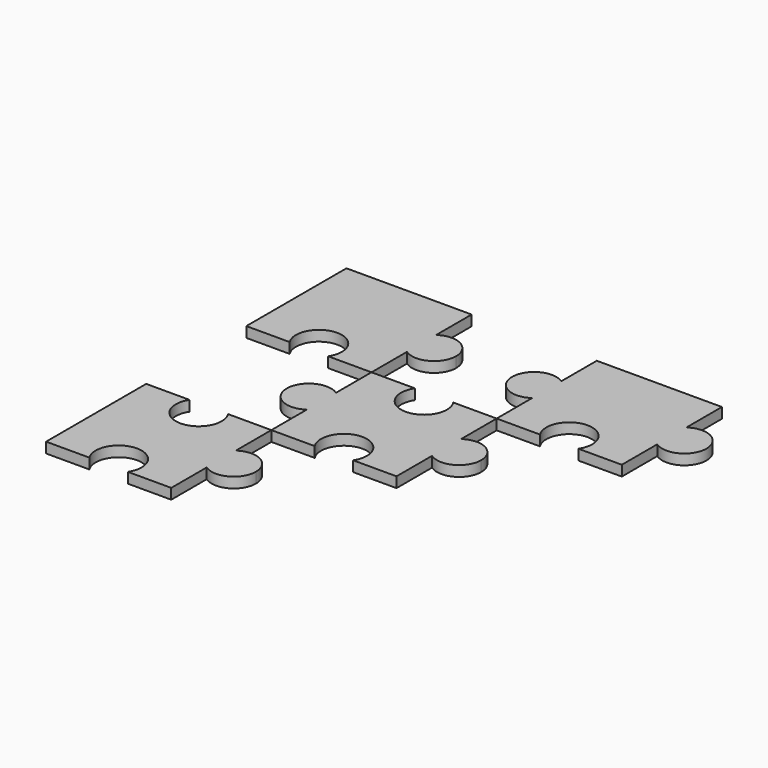
from build123d import *

# Parameters (mm, degrees)
F1_DEPTH = 2.5
F2_DEPTH = 2.5
F3_DEPTH = 2.5
F4_DEPTH = 2.5
F5_ANGLE = 45
F7_ANGLE = -45


# Not quite as in the source:
# - a pattern or mirror of a feature is missing from the dataset's text; its kind, count and spacing are read off the source's solid
# - a feature names something its author has since deleted; it is built from what else it names


with BuildPart() as f1:
    # F0 (on Top) → F1 (new body)
    with BuildSketch(Plane.XY):
        with BuildLine():
            Line((15, 4.6097722286), (15, 15))
            Line((15, 15), (4.6097722286, 15))
            ThreePointArc((4.6097722286, 15), (5.2727482046, 13.564648961), (5.5, 12))
            ThreePointArc((5.5, 12), (-1.564648961, 6.7272517954), (-4.6097722286, 15))
            Line((-4.6097722286, 15), (-15, 15))
            Line((-15, 15), (-15, 4.6097722286))
            ThreePointArc((-15, 4.6097722286), (-9.3779778796, 4.8347699015), (-6.5, 0))
            ThreePointArc((-6.5, 0), (-9.3779778796, -4.8347699015), (-15, -4.6097722286))
            Line((-15, -4.6097722286), (-15, -15))
            Line((-15, -15), (-4.6097722286, -15))
            ThreePointArc((-4.6097722286, -15), (-1.564648961, -6.7272517954), (5.5, -12))
            ThreePointArc((5.5, -12), (5.2727482046, -13.564648961), (4.6097722286, -15))
            Line((4.6097722286, -15), (15, -15))
            Line((15, -15), (15, -4.6097722286))
            ThreePointArc((15, -4.6097722286), (6.5, 0), (15, 4.6097722286))
        make_face()
        with BuildLine():
            ThreePointArc((5.5, 12), (5.2727482046, 13.564648961), (4.6097722286, 15))
            Line((4.6097722286, 15), (4.369210455, 15))
            ThreePointArc((4.369210455, 15), (5.0619569048, 13.5705388547), (5.3, 12))
            ThreePointArc((5.3, 12), (-1.5705388547, 6.9380430952), (-4.369210455, 15))
            Line((-4.369210455, 15), (-4.6097722286, 15))
            ThreePointArc((-4.6097722286, 15), (-1.564648961, 6.7272517954), (5.5, 12))
        make_face()
        with BuildLine():
            ThreePointArc((15.18, 4.4874937326), (15.0893990769, 4.4292665608), (15, 4.369210455))
            ThreePointArc((15, 4.369210455), (16.6898827277, 2.4688053791), (17.3, 0))
            ThreePointArc((17.3, 0), (16.6898827277, -2.4688053791), (15, -4.369210455))
            ThreePointArc((15, -4.369210455), (15.0893990769, -4.4292665608), (15.18, -4.4874937326))
            ThreePointArc((15.18, -4.4874937326), (16.8856934001, -2.5258661881), (17.5, 0))
            ThreePointArc((17.5, 0), (16.8856934001, 2.5258661881), (15.18, 4.4874937326))
        make_face()
        with BuildLine():
            ThreePointArc((-6.7, 0), (-9.5311946209, 4.6898827277), (-15, 4.369210455))
            Line((-15, 4.369210455), (-15, -4.369210455))
            ThreePointArc((-15, -4.369210455), (-9.5311946209, -4.6898827277), (-6.7, 0))
        make_face()
        with BuildLine():
            ThreePointArc((5.3, 12), (5.0619569048, 13.5705388547), (4.369210455, 15))
            Line((4.369210455, 15), (-4.369210455, 15))
            ThreePointArc((-4.369210455, 15), (-1.5705388547, 6.9380430952), (5.3, 12))
        make_face()
        with BuildLine():
            ThreePointArc((14.82, -4.4874937326), (12.5, 0), (14.82, 4.4874937326))
            ThreePointArc((14.82, 4.4874937326), (6.7, 0), (14.82, -4.4874937326))
        make_face()
        with BuildLine():
            Line((15, -4.369210455), (15, 4.369210455))
            ThreePointArc((15, 4.369210455), (12.7, 0), (15, -4.369210455))
        make_face()
        with BuildLine():
            ThreePointArc((17.3, 0), (16.6898827277, 2.4688053791), (15, 4.369210455))
            Line((15, 4.369210455), (15, -4.369210455))
            ThreePointArc((15, -4.369210455), (16.6898827277, -2.4688053791), (17.3, 0))
        make_face()
        with BuildLine():
            ThreePointArc((23.3, 0), (20.5635912311, 4.6387498316), (15.18, 4.4874937326))
            ThreePointArc((15.18, 4.4874937326), (16.8856934001, 2.5258661881), (17.5, 0))
            ThreePointArc((17.5, 0), (16.8856934001, -2.5258661881), (15.18, -4.4874937326))
            ThreePointArc((15.18, -4.4874937326), (20.5635912311, -4.6387498316), (23.3, 0))
        make_face()
        with BuildLine():
            ThreePointArc((15, -4.369210455), (12.7, 0), (15, 4.369210455))
            ThreePointArc((15, 4.369210455), (14.9106009231, 4.4292665608), (14.82, 4.4874937326))
            ThreePointArc((14.82, 4.4874937326), (12.5, 0), (14.82, -4.4874937326))
            ThreePointArc((14.82, -4.4874937326), (14.9106009231, -4.4292665608), (15, -4.369210455))
        make_face()
        with BuildLine():
            ThreePointArc((-6.5, 0), (-9.3779778796, 4.8347699015), (-15, 4.6097722286))
            Line((-15, 4.6097722286), (-15, 4.369210455))
            ThreePointArc((-15, 4.369210455), (-9.5311946209, 4.6898827277), (-6.7, 0))
            ThreePointArc((-6.7, 0), (-9.5311946209, -4.6898827277), (-15, -4.369210455))
            Line((-15, -4.369210455), (-15, -4.6097722286))
            ThreePointArc((-15, -4.6097722286), (-9.3779778796, -4.8347699015), (-6.5, 0))
        make_face()
        with BuildLine():
            ThreePointArc((14.82, 4.4874937326), (14.9093952036, 4.5495232709), (15, 4.6097722286))
            ThreePointArc((15, 4.6097722286), (6.5, 0), (15, -4.6097722286))
            ThreePointArc((15, -4.6097722286), (14.9093952036, -4.5495232709), (14.82, -4.4874937326))
            ThreePointArc((14.82, -4.4874937326), (6.7, 0), (14.82, 4.4874937326))
        make_face()
        with BuildLine():
            Line((15, 4.369210455), (15, 4.6097722286))
            ThreePointArc((15, 4.6097722286), (14.9093952036, 4.5495232709), (14.82, 4.4874937326))
            ThreePointArc((14.82, 4.4874937326), (14.9106009231, 4.4292665608), (15, 4.369210455))
        make_face()
        with BuildLine():
            ThreePointArc((14.82, -4.4874937326), (14.9093952036, -4.5495232709), (15, -4.6097722286))
            Line((15, -4.6097722286), (15, -4.369210455))
            ThreePointArc((15, -4.369210455), (14.9106009231, -4.4292665608), (14.82, -4.4874937326))
        make_face()
    extrude(amount=F1_DEPTH)


with BuildPart() as f2:
    # F0 (on Top) → F2 (new body)
    with BuildSketch(Plane.XY):
        with BuildLine():
            ThreePointArc((44.82, -4.4874937326), (42.5, 0), (44.82, 4.4874937326))
            ThreePointArc((44.82, 4.4874937326), (36.7, 0), (44.82, -4.4874937326))
        make_face()
        with BuildLine():
            Line((45, -4.369210455), (45, 4.369210455))
            ThreePointArc((45, 4.369210455), (42.7, 0), (45, -4.369210455))
        make_face()
        with BuildLine():
            ThreePointArc((45, -4.369210455), (42.7, 0), (45, 4.369210455))
            ThreePointArc((45, 4.369210455), (44.9106009231, 4.4292665608), (44.82, 4.4874937326))
            ThreePointArc((44.82, 4.4874937326), (42.5, 0), (44.82, -4.4874937326))
            ThreePointArc((44.82, -4.4874937326), (44.9106009231, -4.4292665608), (45, -4.369210455))
        make_face()
        with BuildLine():
            ThreePointArc((47.3, 0), (46.6898827277, 2.4688053791), (45, 4.369210455))
            Line((45, 4.369210455), (45, -4.369210455))
            ThreePointArc((45, -4.369210455), (46.6898827277, -2.4688053791), (47.3, 0))
        make_face()
        with BuildLine():
            ThreePointArc((47.5, 0), (46.8856934001, 2.5258661881), (45.18, 4.4874937326))
            ThreePointArc((45.18, 4.4874937326), (45.0893990769, 4.4292665608), (45, 4.369210455))
            ThreePointArc((45, 4.369210455), (46.6898827277, 2.4688053791), (47.3, 0))
            ThreePointArc((47.3, 0), (46.6898827277, -2.4688053791), (45, -4.369210455))
            ThreePointArc((45, -4.369210455), (45.0893990769, -4.4292665608), (45.18, -4.4874937326))
            ThreePointArc((45.18, -4.4874937326), (46.8856934001, -2.5258661881), (47.5, 0))
        make_face()
        with BuildLine():
            ThreePointArc((53.3, 0), (50.5635912311, 4.6387498316), (45.18, 4.4874937326))
            ThreePointArc((45.18, 4.4874937326), (46.8856934001, 2.5258661881), (47.5, 0))
            ThreePointArc((47.5, 0), (46.8856934001, -2.5258661881), (45.18, -4.4874937326))
            ThreePointArc((45.18, -4.4874937326), (50.5635912311, -4.6387498316), (53.3, 0))
        make_face()
        with BuildLine():
            ThreePointArc((53.5, 0), (50.6220221204, 4.8347699015), (45, 4.6097722286))
            ThreePointArc((45, 4.6097722286), (45.0906047964, 4.5495232709), (45.18, 4.4874937326))
            ThreePointArc((45.18, 4.4874937326), (50.5635912311, 4.6387498316), (53.3, 0))
            ThreePointArc((53.3, 0), (50.5635912311, -4.6387498316), (45.18, -4.4874937326))
            ThreePointArc((45.18, -4.4874937326), (45.0906047964, -4.5495232709), (45, -4.6097722286))
            ThreePointArc((45, -4.6097722286), (50.6220221204, -4.8347699015), (53.5, 0))
        make_face()
        with BuildLine():
            Line((55.3902277714, 15), (45, 15))
            Line((45, 15), (45, 4.6097722286))
            ThreePointArc((45, 4.6097722286), (50.6220221204, 4.8347699015), (53.5, 0))
            ThreePointArc((53.5, 0), (50.6220221204, -4.8347699015), (45, -4.6097722286))
            Line((45, -4.6097722286), (45, -15))
            Line((45, -15), (55.3902277714, -15))
            ThreePointArc((55.3902277714, -15), (58.435351039, -6.7272517954), (65.5, -12))
            ThreePointArc((65.5, -12), (65.2727482046, -13.564648961), (64.6097722286, -15))
            Line((64.6097722286, -15), (75, -15))
            Line((75, -15), (75, -4.6097722286))
            ThreePointArc((75, -4.6097722286), (66.5, 0), (75, 4.6097722286))
            Line((75, 4.6097722286), (75, 15))
            Line((75, 15), (64.6097722286, 15))
            ThreePointArc((64.6097722286, 15), (65.2727482046, 13.564648961), (65.5, 12))
            ThreePointArc((65.5, 12), (58.435351039, 6.7272517954), (55.3902277714, 15))
        make_face()
        with BuildLine():
            ThreePointArc((45.18, 4.4874937326), (45.0906047964, 4.5495232709), (45, 4.6097722286))
            Line((45, 4.6097722286), (45, 4.369210455))
            ThreePointArc((45, 4.369210455), (45.0893990769, 4.4292665608), (45.18, 4.4874937326))
        make_face()
        with BuildLine():
            Line((45, -4.369210455), (45, -4.6097722286))
            ThreePointArc((45, -4.6097722286), (45.0906047964, -4.5495232709), (45.18, -4.4874937326))
            ThreePointArc((45.18, -4.4874937326), (45.0893990769, -4.4292665608), (45, -4.369210455))
        make_face()
        with BuildLine():
            Line((64.369210455, 15), (55.630789545, 15))
            ThreePointArc((55.630789545, 15), (58.4294611453, 6.9380430952), (65.3, 12))
            ThreePointArc((65.3, 12), (65.0619569048, 13.5705388547), (64.369210455, 15))
        make_face()
        with BuildLine():
            Line((55.630789545, 15), (55.3902277714, 15))
            ThreePointArc((55.3902277714, 15), (58.435351039, 6.7272517954), (65.5, 12))
            ThreePointArc((65.5, 12), (65.2727482046, 13.564648961), (64.6097722286, 15))
            Line((64.6097722286, 15), (64.369210455, 15))
            ThreePointArc((64.369210455, 15), (65.0619569048, 13.5705388547), (65.3, 12))
            ThreePointArc((65.3, 12), (58.4294611453, 6.9380430952), (55.630789545, 15))
        make_face()
    extrude(amount=F2_DEPTH)



with BuildPart() as f2b:
    # F0 (on Top) → F2, piece 2 (new body)
    with BuildSketch(Plane.XY):
        with BuildLine():
            ThreePointArc((77.3, 0), (76.6898827277, 2.4688053791), (75, 4.369210455))
            Line((75, 4.369210455), (75, -4.369210455))
            ThreePointArc((75, -4.369210455), (76.6898827277, -2.4688053791), (77.3, 0))
        make_face()
        with BuildLine():
            Line((75, -4.369210455), (75, 4.369210455))
            ThreePointArc((75, 4.369210455), (72.7, 0), (75, -4.369210455))
        make_face()
    extrude(amount=F2_DEPTH)


with BuildPart() as f2_1:
    add(f2.part)

    add(f2b.part)  # F2_copies merges F2b
    # F2_copies: F2 across plane
    add(f2.part.mirror(Plane(origin=(60, 0, 0), x_dir=(0, 0, 1), z_dir=(1, 0, 0))))


with BuildPart() as f3:
    # F0 (on Top) → F3 (new body)
    with BuildSketch(Plane.XY):
        with BuildLine():
            Line((15, -55.3902277714), (15, -45))
            Line((15, -45), (4.6097722286, -45))
            ThreePointArc((4.6097722286, -45), (5.2727482046, -46.435351039), (5.5, -48))
            ThreePointArc((5.5, -48), (-1.564648961, -53.2727482046), (-4.6097722286, -45))
            Line((-4.6097722286, -45), (-15, -45))
            Line((-15, -45), (-15, -55.3902277714))
            ThreePointArc((-15, -55.3902277714), (-9.3779778796, -55.1652300985), (-6.5, -60))
            ThreePointArc((-6.5, -60), (-9.3779778796, -64.8347699015), (-15, -64.6097722286))
            Line((-15, -64.6097722286), (-15, -75))
            Line((-15, -75), (-4.6097722286, -75))
            ThreePointArc((-4.6097722286, -75), (-1.564648961, -66.7272517954), (5.5, -72))
            ThreePointArc((5.5, -72), (5.2727482046, -73.564648961), (4.6097722286, -75))
            Line((4.6097722286, -75), (15, -75))
            Line((15, -75), (15, -64.6097722286))
            ThreePointArc((15, -64.6097722286), (6.5, -60), (15, -55.3902277714))
        make_face()
        with BuildLine():
            ThreePointArc((-6.7, -60), (-9.5311946209, -55.3101172723), (-15, -55.630789545))
            Line((-15, -55.630789545), (-15, -64.369210455))
            ThreePointArc((-15, -64.369210455), (-9.5311946209, -64.6898827277), (-6.7, -60))
        make_face()
        with BuildLine():
            ThreePointArc((14.82, -64.4874937326), (12.5, -60), (14.82, -55.5125062674))
            ThreePointArc((14.82, -55.5125062674), (6.7, -60), (14.82, -64.4874937326))
        make_face()
        with BuildLine():
            ThreePointArc((23.3, -60), (20.5635912311, -55.3612501684), (15.18, -55.5125062674))
            ThreePointArc((15.18, -55.5125062674), (16.8856934001, -57.4741338119), (17.5, -60))
            ThreePointArc((17.5, -60), (16.8856934001, -62.5258661881), (15.18, -64.4874937326))
            ThreePointArc((15.18, -64.4874937326), (20.5635912311, -64.6387498316), (23.3, -60))
        make_face()
        with BuildLine():
            ThreePointArc((17.3, -60), (16.6898827277, -57.5311946209), (15, -55.630789545))
            Line((15, -55.630789545), (15, -64.369210455))
            ThreePointArc((15, -64.369210455), (16.6898827277, -62.4688053791), (17.3, -60))
        make_face()
        with BuildLine():
            Line((15, -64.369210455), (15, -55.630789545))
            ThreePointArc((15, -55.630789545), (12.7, -60), (15, -64.369210455))
        make_face()
        with BuildLine():
            ThreePointArc((-6.5, -60), (-9.3779778796, -55.1652300985), (-15, -55.3902277714))
            Line((-15, -55.3902277714), (-15, -55.630789545))
            ThreePointArc((-15, -55.630789545), (-9.5311946209, -55.3101172723), (-6.7, -60))
            ThreePointArc((-6.7, -60), (-9.5311946209, -64.6898827277), (-15, -64.369210455))
            Line((-15, -64.369210455), (-15, -64.6097722286))
            ThreePointArc((-15, -64.6097722286), (-9.3779778796, -64.8347699015), (-6.5, -60))
        make_face()
        with BuildLine():
            ThreePointArc((14.82, -55.5125062674), (14.9093952036, -55.4504767291), (15, -55.3902277714))
            ThreePointArc((15, -55.3902277714), (6.5, -60), (15, -64.6097722286))
            ThreePointArc((15, -64.6097722286), (14.9093952036, -64.5495232709), (14.82, -64.4874937326))
            ThreePointArc((14.82, -64.4874937326), (6.7, -60), (14.82, -55.5125062674))
        make_face()
        with BuildLine():
            ThreePointArc((15, -64.369210455), (12.7, -60), (15, -55.630789545))
            ThreePointArc((15, -55.630789545), (14.9106009231, -55.5707334392), (14.82, -55.5125062674))
            ThreePointArc((14.82, -55.5125062674), (12.5, -60), (14.82, -64.4874937326))
            ThreePointArc((14.82, -64.4874937326), (14.9106009231, -64.4292665608), (15, -64.369210455))
        make_face()
        with BuildLine():
            ThreePointArc((17.5, -60), (16.8856934001, -57.4741338119), (15.18, -55.5125062674))
            ThreePointArc((15.18, -55.5125062674), (15.0893990769, -55.5707334392), (15, -55.630789545))
            ThreePointArc((15, -55.630789545), (16.6898827277, -57.5311946209), (17.3, -60))
            ThreePointArc((17.3, -60), (16.6898827277, -62.4688053791), (15, -64.369210455))
            ThreePointArc((15, -64.369210455), (15.0893990769, -64.4292665608), (15.18, -64.4874937326))
            ThreePointArc((15.18, -64.4874937326), (16.8856934001, -62.5258661881), (17.5, -60))
        make_face()
        with BuildLine():
            Line((15, -55.630789545), (15, -55.3902277714))
            ThreePointArc((15, -55.3902277714), (14.9093952036, -55.4504767291), (14.82, -55.5125062674))
            ThreePointArc((14.82, -55.5125062674), (14.9106009231, -55.5707334392), (15, -55.630789545))
        make_face()
        with BuildLine():
            ThreePointArc((14.82, -64.4874937326), (14.9093952036, -64.5495232709), (15, -64.6097722286))
            Line((15, -64.6097722286), (15, -64.369210455))
            ThreePointArc((15, -64.369210455), (14.9106009231, -64.4292665608), (14.82, -64.4874937326))
        make_face()
    extrude(amount=F3_DEPTH)


with BuildPart() as f4:
    # F0 (on Top) → F4 (new body)
    with BuildSketch(Plane.XY):
        with BuildLine():
            ThreePointArc((14.82, -34.4874937326), (12.5, -30), (14.82, -25.5125062674))
            ThreePointArc((14.82, -25.5125062674), (6.7, -30), (14.82, -34.4874937326))
        make_face()
        with BuildLine():
            Line((25.3902277714, -15), (15, -15))
            Line((15, -15), (15, -25.3902277714))
            ThreePointArc((15, -25.3902277714), (20.6220221204, -25.1652300985), (23.5, -30))
            ThreePointArc((23.5, -30), (20.6220221204, -34.8347699015), (15, -34.6097722286))
            Line((15, -34.6097722286), (15, -45))
            Line((15, -45), (25.3902277714, -45))
            ThreePointArc((25.3902277714, -45), (28.435351039, -36.7272517954), (35.5, -42))
            ThreePointArc((35.5, -42), (35.2727482046, -43.564648961), (34.6097722286, -45))
            Line((34.6097722286, -45), (45, -45))
            Line((45, -45), (45, -34.6097722286))
            ThreePointArc((45, -34.6097722286), (36.5, -30), (45, -25.3902277714))
            Line((45, -25.3902277714), (45, -15))
            Line((45, -15), (34.6097722286, -15))
            ThreePointArc((34.6097722286, -15), (35.2727482046, -16.435351039), (35.5, -18))
            ThreePointArc((35.5, -18), (28.435351039, -23.2727482046), (25.3902277714, -15))
        make_face()
        with BuildLine():
            ThreePointArc((23.3, -30), (20.5635912311, -25.3612501684), (15.18, -25.5125062674))
            ThreePointArc((15.18, -25.5125062674), (16.8856934001, -27.4741338119), (17.5, -30))
            ThreePointArc((17.5, -30), (16.8856934001, -32.5258661881), (15.18, -34.4874937326))
            ThreePointArc((15.18, -34.4874937326), (20.5635912311, -34.6387498316), (23.3, -30))
        make_face()
        with BuildLine():
            ThreePointArc((17.3, -30), (16.6898827277, -27.5311946209), (15, -25.630789545))
            Line((15, -25.630789545), (15, -34.369210455))
            ThreePointArc((15, -34.369210455), (16.6898827277, -32.4688053791), (17.3, -30))
        make_face()
        with BuildLine():
            Line((15, -34.369210455), (15, -25.630789545))
            ThreePointArc((15, -25.630789545), (12.7, -30), (15, -34.369210455))
        make_face()
        with BuildLine():
            ThreePointArc((53.3, -30), (50.5635912311, -25.3612501684), (45.18, -25.5125062674))
            ThreePointArc((45.18, -25.5125062674), (46.8856934001, -27.4741338119), (47.5, -30))
            ThreePointArc((47.5, -30), (46.8856934001, -32.5258661881), (45.18, -34.4874937326))
            ThreePointArc((45.18, -34.4874937326), (50.5635912311, -34.6387498316), (53.3, -30))
        make_face()
        with BuildLine():
            ThreePointArc((47.3, -30), (46.6898827277, -27.5311946209), (45, -25.630789545))
            Line((45, -25.630789545), (45, -34.369210455))
            ThreePointArc((45, -34.369210455), (46.6898827277, -32.4688053791), (47.3, -30))
        make_face()
        with BuildLine():
            Line((45, -34.369210455), (45, -25.630789545))
            ThreePointArc((45, -25.630789545), (42.7, -30), (45, -34.369210455))
        make_face()
        with BuildLine():
            ThreePointArc((44.82, -34.4874937326), (42.5, -30), (44.82, -25.5125062674))
            ThreePointArc((44.82, -25.5125062674), (36.7, -30), (44.82, -34.4874937326))
        make_face()
        with BuildLine():
            ThreePointArc((17.5, -30), (16.8856934001, -27.4741338119), (15.18, -25.5125062674))
            ThreePointArc((15.18, -25.5125062674), (15.0893990769, -25.5707334392), (15, -25.630789545))
            ThreePointArc((15, -25.630789545), (16.6898827277, -27.5311946209), (17.3, -30))
            ThreePointArc((17.3, -30), (16.6898827277, -32.4688053791), (15, -34.369210455))
            ThreePointArc((15, -34.369210455), (15.0893990769, -34.4292665608), (15.18, -34.4874937326))
            ThreePointArc((15.18, -34.4874937326), (16.8856934001, -32.5258661881), (17.5, -30))
        make_face()
        with BuildLine():
            ThreePointArc((15, -34.369210455), (12.7, -30), (15, -25.630789545))
            ThreePointArc((15, -25.630789545), (14.9106009231, -25.5707334392), (14.82, -25.5125062674))
            ThreePointArc((14.82, -25.5125062674), (12.5, -30), (14.82, -34.4874937326))
            ThreePointArc((14.82, -34.4874937326), (14.9106009231, -34.4292665608), (15, -34.369210455))
        make_face()
        with BuildLine():
            ThreePointArc((23.5, -30), (20.6220221204, -25.1652300985), (15, -25.3902277714))
            ThreePointArc((15, -25.3902277714), (15.0906047964, -25.4504767291), (15.18, -25.5125062674))
            ThreePointArc((15.18, -25.5125062674), (20.5635912311, -25.3612501684), (23.3, -30))
            ThreePointArc((23.3, -30), (20.5635912311, -34.6387498316), (15.18, -34.4874937326))
            ThreePointArc((15.18, -34.4874937326), (15.0906047964, -34.5495232709), (15, -34.6097722286))
            ThreePointArc((15, -34.6097722286), (20.6220221204, -34.8347699015), (23.5, -30))
        make_face()
        with BuildLine():
            ThreePointArc((15.18, -25.5125062674), (15.0906047964, -25.4504767291), (15, -25.3902277714))
            Line((15, -25.3902277714), (15, -25.630789545))
            ThreePointArc((15, -25.630789545), (15.0893990769, -25.5707334392), (15.18, -25.5125062674))
        make_face()
        with BuildLine():
            Line((15, -34.369210455), (15, -34.6097722286))
            ThreePointArc((15, -34.6097722286), (15.0906047964, -34.5495232709), (15.18, -34.4874937326))
            ThreePointArc((15.18, -34.4874937326), (15.0893990769, -34.4292665608), (15, -34.369210455))
        make_face()
        with BuildLine():
            ThreePointArc((44.82, -25.5125062674), (44.9093952036, -25.4504767291), (45, -25.3902277714))
            ThreePointArc((45, -25.3902277714), (36.5, -30), (45, -34.6097722286))
            ThreePointArc((45, -34.6097722286), (44.9093952036, -34.5495232709), (44.82, -34.4874937326))
            ThreePointArc((44.82, -34.4874937326), (36.7, -30), (44.82, -25.5125062674))
        make_face()
        with BuildLine():
            ThreePointArc((44.82, -34.4874937326), (44.9093952036, -34.5495232709), (45, -34.6097722286))
            Line((45, -34.6097722286), (45, -34.369210455))
            ThreePointArc((45, -34.369210455), (44.9106009231, -34.4292665608), (44.82, -34.4874937326))
        make_face()
        with BuildLine():
            ThreePointArc((45, -34.369210455), (42.7, -30), (45, -25.630789545))
            ThreePointArc((45, -25.630789545), (44.9106009231, -25.5707334392), (44.82, -25.5125062674))
            ThreePointArc((44.82, -25.5125062674), (42.5, -30), (44.82, -34.4874937326))
            ThreePointArc((44.82, -34.4874937326), (44.9106009231, -34.4292665608), (45, -34.369210455))
        make_face()
        with BuildLine():
            ThreePointArc((47.5, -30), (46.8856934001, -27.4741338119), (45.18, -25.5125062674))
            ThreePointArc((45.18, -25.5125062674), (45.0893990769, -25.5707334392), (45, -25.630789545))
            ThreePointArc((45, -25.630789545), (46.6898827277, -27.5311946209), (47.3, -30))
            ThreePointArc((47.3, -30), (46.6898827277, -32.4688053791), (45, -34.369210455))
            ThreePointArc((45, -34.369210455), (45.0893990769, -34.4292665608), (45.18, -34.4874937326))
            ThreePointArc((45.18, -34.4874937326), (46.8856934001, -32.5258661881), (47.5, -30))
        make_face()
        with BuildLine():
            Line((45, -25.630789545), (45, -25.3902277714))
            ThreePointArc((45, -25.3902277714), (44.9093952036, -25.4504767291), (44.82, -25.5125062674))
            ThreePointArc((44.82, -25.5125062674), (44.9106009231, -25.5707334392), (45, -25.630789545))
        make_face()
    extrude(amount=F4_DEPTH)


with BuildPart() as f1_1:
    # F5: moved
    add(f1.part.rotate(Axis((-4.6097722286, -15, 1.25), (0, 0, -1)), F5_ANGLE))


with BuildPart() as f2_2:
    # F5: moved
    add(f2_1.part.rotate(Axis((-4.6097722286, -15, 1.25), (0, 0, -1)), F5_ANGLE))


with BuildPart() as f4_1:
    # F5: moved
    add(f4.part.rotate(Axis((-4.6097722286, -15, 1.25), (0, 0, -1)), F5_ANGLE))


with BuildPart() as f3_1:
    # F5: moved
    add(f3.part.rotate(Axis((-4.6097722286, -15, 1.25), (0, 0, -1)), F5_ANGLE))


with BuildPart() as f1_2:
    # F7: moved
    add(f1_1.part.rotate(Axis((-4.6097722286, -15, 1.25), (0, 0, -1)), F7_ANGLE))


with BuildPart() as f2_3:
    # F7: moved
    add(f2_2.part.rotate(Axis((-4.6097722286, -15, 1.25), (0, 0, -1)), F7_ANGLE))


with BuildPart() as f3_2:
    # F7: moved
    add(f3_1.part.rotate(Axis((-4.6097722286, -15, 1.25), (0, 0, -1)), F7_ANGLE))


with BuildPart() as f4_2:
    # F7: moved
    add(f4_1.part.rotate(Axis((-4.6097722286, -15, 1.25), (0, 0, -1)), F7_ANGLE))


solid = Compound([f1_2.part, f2_3.part, f3_2.part, f4_2.part])
